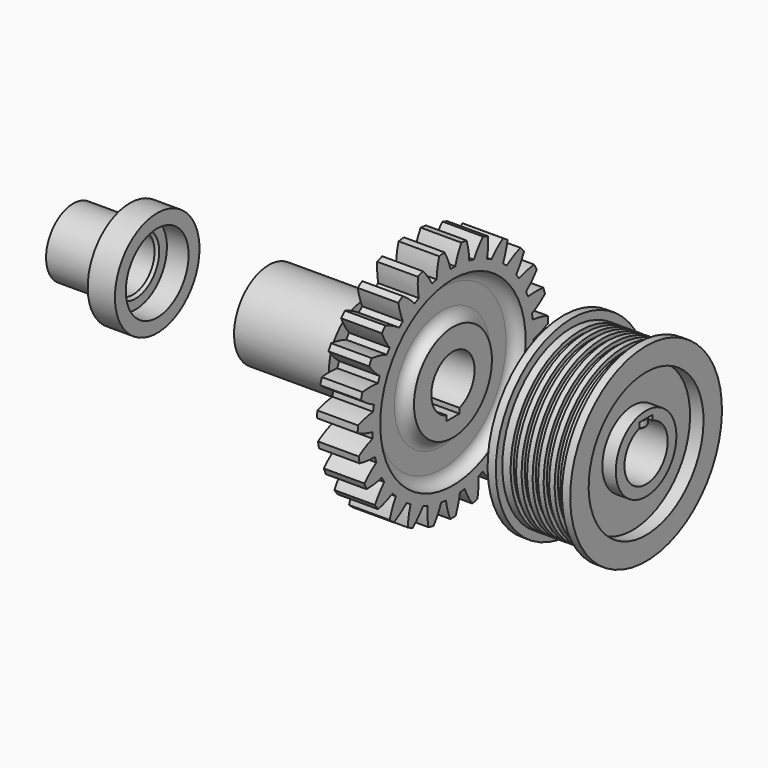
from build123d import *

# Parameters (mm, degrees)
F3_DEPTH  = 127
F7_DEPTH  = 45.212
F10_DEPTH = 39.878
F11_SIZE  = 2.032
F12_R     = 5.96899
F16_DEPTH = 33.02
F17_COUNT = 27
F17_ANGLE = 346.6666666667
F20_DEPTH = 33.02
F22_W     = 70.104
F22_H     = 12.065
F26_SIZE  = 1.905
F29_DEPTH = 6.096
F30_SIZE  = 0.762


# Not quite as in the source:
# - a fillet or chamfer that OpenCascade refuses, or shapes differently, is made with other operations: its cross-section is extruded or revolved along the edge and cut away or added
# - a fillet or chamfer is up to 0.001 mm smaller than in the source, because OpenCascade refuses the exact size


with BuildPart() as f1:
    # F0 (on Front) → F1 (revolve)
    with BuildSketch(Plane.XZ):
        Polygon((-30.48, 69.977), (-30.48, 52.959), (-20.574, 52.959), (-20.574, 27.94), (-30.48, 27.94), (-30.48, 19.939), (30.48, 19.939), (30.48, 27.94), (20.574, 27.94), (20.574, 52.959), (30.48, 52.959), (30.48, 69.977), (24.384, 69.977), (24.384, 64.008), (18.288, 64.008), (18.288, 60.96), (14.224, 60.96), (14.224, 64.008), (10.16, 64.008), (10.16, 60.96), (6.096, 60.96), (6.096, 64.008), (2.032, 64.008), (2.032, 60.96), (-2.032, 60.96), (-2.032, 64.008), (-6.096, 64.008), (-6.096, 60.96), (-10.16, 60.96), (-10.16, 64.008), (-14.224, 64.008), (-14.224, 60.96), (-18.288, 60.96), (-18.288, 64.008), (-24.384, 64.008), (-24.384, 69.977), align=None)
    revolve(axis=Axis((0, 0, 0), (1, 0, 0)))

    # F2 (on face) → F3 (cut)
    with BuildSketch(Plane(origin=(-30.48, 0, 0), x_dir=(0, -1, 0), z_dir=(-1, 0, 0))):
        with BuildLine():
            Line((5.969, 22.8345830441), (-5.969, 22.8345830441))
            Line((-5.969, 22.8345830441), (-5.969, 19.0245830441))
            ThreePointArc((-5.969, 19.0245830441), (0, 19.939), (5.969, 19.0245830441))
            Line((5.969, 19.0245830441), (5.969, 22.8345830441))
        make_face()
    extrude(amount=-F3_DEPTH, mode=Mode.SUBTRACT)


with BuildPart() as f5:
    # F4 (on Front) → F5 (revolve)
    with BuildSketch(Plane.XZ):
        Polygon((623.316, 19.939), (43.18, 19.939), (43.18, 0), (1083.056, 0), (1083.056, 19.939), (1003.3, 19.939), (1003.3, 28.956), (988.314, 28.956), (988.314, 19.939), (638.302, 19.939), (638.302, 28.956), (623.316, 28.956), align=None)
    revolve(axis=Axis((563.118, 0, 0), (1, 0, 0)))

    # F6 (on face) → F7 (cut)
    with BuildSketch(Plane(origin=(43.18, 0, 0), x_dir=(0, -1, 0), z_dir=(-1, 0, 0))):
        with BuildLine():
            ThreePointArc((5.969, 19.0245830441), (0, 19.939), (-5.969, 19.0245830441))
            Line((-5.969, 19.0245830441), (-5.969, 16.4845830441))
            Line((-5.969, 16.4845830441), (5.969, 16.4845830441))
            Line((5.969, 16.4845830441), (5.969, 19.0245830441))
        make_face()
    extrude(amount=-F7_DEPTH, mode=Mode.SUBTRACT)

    # F9 (on offset) → F10 (cut)
    with BuildSketch(Plane(origin=(585.216, 0, 0), x_dir=(0, -1, 0), z_dir=(-1, 0, 0))):
        with BuildLine():
            ThreePointArc((5.969, 19.0245830441), (0, 19.939), (-5.969, 19.0245830441))
            Line((-5.969, 19.0245830441), (-5.969, 16.4845830441))
            Line((-5.969, 16.4845830441), (5.969, 16.4845830441))
            Line((5.969, 16.4845830441), (5.969, 19.0245830441))
        make_face()
    extrude(amount=F10_DEPTH, mode=Mode.SUBTRACT)

    # F11
    f11_edges = [f5.edges().sort_by_distance(p)[0] for p in [
        (43.18, 0, -19.939),
        (1083.056, 0, -19.939),
    ]]
    chamfer(f11_edges, length=F11_SIZE)

    # F12 (radius 5.969 in the source; OpenCascade refuses exactly that, so slightly less here)
    f12_edges = [f5.edges().sort_by_distance(p)[0] for p in [
        (585.216, 5.969, 17.754583),
        (585.216, -5.969, 17.754583),
        (545.338, 5.969, 17.754583),
        (545.338, -5.969, 17.754583),
        (88.392, 5.969, 17.754583),
        (88.392, -5.969, 17.754583),
    ]]
    fillet(f12_edges, radius=F12_R)


with BuildPart() as f14:
    # F13 (on Front) → F14 (revolve)
    with BuildSketch(Plane.XZ):
        Polygon((-141.986, 35.941), (-141.986, 19.939), (-112.014, 19.939), (-112.014, 35.941), (-120.015, 35.941), (-120.015, 67.056), (-112.014, 67.056), (-112.014, 87.884), (-141.986, 87.884), (-141.986, 67.056), (-133.985, 67.056), (-133.985, 35.941), align=None)
    revolve(axis=Axis((-127, 0, 0), (1, 0, 0)))


with BuildPart() as f16:
    # F15 (on face) → F16 (new body)
    with BuildSketch(Plane(origin=(-141.986, 0, 0), x_dir=(0, -1, 0), z_dir=(-1, 0, 0))):
        with BuildLine():
            ThreePointArc((-7.747, 87.5418839585), (-4.5366280447, 81.1431985003), (-2.159, 74.3906768554))
            ThreePointArc((-2.159, 74.3906768554), (0, 74.422), (2.159, 74.3906768554))
            ThreePointArc((2.159, 74.3906768554), (4.5366280447, 81.1431985003), (7.747, 87.5418839585))
            ThreePointArc((7.747, 87.5418839585), (0, 87.884), (-7.747, 87.5418839585))
        make_face()
    extrude(amount=-F16_DEPTH)


with BuildPart() as f17_1:
    # F17: instance of F16
    add(f16.part.rotate(Axis((-141.986, 0, 0), (1, 0, 0)), 1 * F17_ANGLE / (F17_COUNT - 1)))


with BuildPart() as f17_2:
    # F17: instance of F16
    add(f16.part.rotate(Axis((-141.986, 0, 0), (1, 0, 0)), 2 * F17_ANGLE / (F17_COUNT - 1)))


with BuildPart() as f17_3:
    # F17: instance of F16
    add(f16.part.rotate(Axis((-141.986, 0, 0), (1, 0, 0)), 3 * F17_ANGLE / (F17_COUNT - 1)))


with BuildPart() as f17_4:
    # F17: instance of F16
    add(f16.part.rotate(Axis((-141.986, 0, 0), (1, 0, 0)), 4 * F17_ANGLE / (F17_COUNT - 1)))


with BuildPart() as f17_5:
    # F17: instance of F16
    add(f16.part.rotate(Axis((-141.986, 0, 0), (1, 0, 0)), 5 * F17_ANGLE / (F17_COUNT - 1)))


with BuildPart() as f17_6:
    # F17: instance of F16
    add(f16.part.rotate(Axis((-141.986, 0, 0), (1, 0, 0)), 6 * F17_ANGLE / (F17_COUNT - 1)))


with BuildPart() as f17_7:
    # F17: instance of F16
    add(f16.part.rotate(Axis((-141.986, 0, 0), (1, 0, 0)), 7 * F17_ANGLE / (F17_COUNT - 1)))


with BuildPart() as f17_8:
    # F17: instance of F16
    add(f16.part.rotate(Axis((-141.986, 0, 0), (1, 0, 0)), 8 * F17_ANGLE / (F17_COUNT - 1)))


with BuildPart() as f17_9:
    # F17: instance of F16
    add(f16.part.rotate(Axis((-141.986, 0, 0), (1, 0, 0)), 9 * F17_ANGLE / (F17_COUNT - 1)))


with BuildPart() as f17_10:
    # F17: instance of F16
    add(f16.part.rotate(Axis((-141.986, 0, 0), (1, 0, 0)), 10 * F17_ANGLE / (F17_COUNT - 1)))


with BuildPart() as f17_11:
    # F17: instance of F16
    add(f16.part.rotate(Axis((-141.986, 0, 0), (1, 0, 0)), 11 * F17_ANGLE / (F17_COUNT - 1)))


with BuildPart() as f17_12:
    # F17: instance of F16
    add(f16.part.rotate(Axis((-141.986, 0, 0), (1, 0, 0)), 12 * F17_ANGLE / (F17_COUNT - 1)))


with BuildPart() as f17_13:
    # F17: instance of F16
    add(f16.part.rotate(Axis((-141.986, 0, 0), (1, 0, 0)), 13 * F17_ANGLE / (F17_COUNT - 1)))


with BuildPart() as f17_14:
    # F17: instance of F16
    add(f16.part.rotate(Axis((-141.986, 0, 0), (1, 0, 0)), 14 * F17_ANGLE / (F17_COUNT - 1)))


with BuildPart() as f17_15:
    # F17: instance of F16
    add(f16.part.rotate(Axis((-141.986, 0, 0), (1, 0, 0)), 15 * F17_ANGLE / (F17_COUNT - 1)))


with BuildPart() as f17_16:
    # F17: instance of F16
    add(f16.part.rotate(Axis((-141.986, 0, 0), (1, 0, 0)), 16 * F17_ANGLE / (F17_COUNT - 1)))


with BuildPart() as f17_17:
    # F17: instance of F16
    add(f16.part.rotate(Axis((-141.986, 0, 0), (1, 0, 0)), 17 * F17_ANGLE / (F17_COUNT - 1)))


with BuildPart() as f17_18:
    # F17: instance of F16
    add(f16.part.rotate(Axis((-141.986, 0, 0), (1, 0, 0)), 18 * F17_ANGLE / (F17_COUNT - 1)))


with BuildPart() as f17_19:
    # F17: instance of F16
    add(f16.part.rotate(Axis((-141.986, 0, 0), (1, 0, 0)), 19 * F17_ANGLE / (F17_COUNT - 1)))


with BuildPart() as f17_20:
    # F17: instance of F16
    add(f16.part.rotate(Axis((-141.986, 0, 0), (1, 0, 0)), 20 * F17_ANGLE / (F17_COUNT - 1)))


with BuildPart() as f17_21:
    # F17: instance of F16
    add(f16.part.rotate(Axis((-141.986, 0, 0), (1, 0, 0)), 21 * F17_ANGLE / (F17_COUNT - 1)))


with BuildPart() as f17_22:
    # F17: instance of F16
    add(f16.part.rotate(Axis((-141.986, 0, 0), (1, 0, 0)), 22 * F17_ANGLE / (F17_COUNT - 1)))


with BuildPart() as f17_23:
    # F17: instance of F16
    add(f16.part.rotate(Axis((-141.986, 0, 0), (1, 0, 0)), 23 * F17_ANGLE / (F17_COUNT - 1)))


with BuildPart() as f17_24:
    # F17: instance of F16
    add(f16.part.rotate(Axis((-141.986, 0, 0), (1, 0, 0)), 24 * F17_ANGLE / (F17_COUNT - 1)))


with BuildPart() as f17_25:
    # F17: instance of F16
    add(f16.part.rotate(Axis((-141.986, 0, 0), (1, 0, 0)), 25 * F17_ANGLE / (F17_COUNT - 1)))


with BuildPart() as f17_26:
    # F17: instance of F16
    add(f16.part.rotate(Axis((-141.986, 0, 0), (1, 0, 0)), 26 * F17_ANGLE / (F17_COUNT - 1)))


with BuildPart() as f14_1:
    add(f14.part)

    # F18: cut F17_26, F16, F17_1, F17_2, F17_3, F17_4, F17_5, F17_6, F17_7, F17_8, F17_25, F17_9, F17_10, F17_11, F17_12, F17_13, F17_14, F17_15, F17_16, F17_17, F17_18, F17_19, F17_20, F17_21, F17_22, F17_23, F17_24
    add(f17_26.part, mode=Mode.SUBTRACT)
    add(f16.part, mode=Mode.SUBTRACT)
    add(f17_1.part, mode=Mode.SUBTRACT)
    add(f17_2.part, mode=Mode.SUBTRACT)
    add(f17_3.part, mode=Mode.SUBTRACT)
    add(f17_4.part, mode=Mode.SUBTRACT)
    add(f17_5.part, mode=Mode.SUBTRACT)
    add(f17_6.part, mode=Mode.SUBTRACT)
    add(f17_7.part, mode=Mode.SUBTRACT)
    add(f17_8.part, mode=Mode.SUBTRACT)
    add(f17_25.part, mode=Mode.SUBTRACT)
    add(f17_9.part, mode=Mode.SUBTRACT)
    add(f17_10.part, mode=Mode.SUBTRACT)
    add(f17_11.part, mode=Mode.SUBTRACT)
    add(f17_12.part, mode=Mode.SUBTRACT)
    add(f17_13.part, mode=Mode.SUBTRACT)
    add(f17_14.part, mode=Mode.SUBTRACT)
    add(f17_15.part, mode=Mode.SUBTRACT)
    add(f17_16.part, mode=Mode.SUBTRACT)
    add(f17_17.part, mode=Mode.SUBTRACT)
    add(f17_18.part, mode=Mode.SUBTRACT)
    add(f17_19.part, mode=Mode.SUBTRACT)
    add(f17_20.part, mode=Mode.SUBTRACT)
    add(f17_21.part, mode=Mode.SUBTRACT)
    add(f17_22.part, mode=Mode.SUBTRACT)
    add(f17_23.part, mode=Mode.SUBTRACT)
    add(f17_24.part, mode=Mode.SUBTRACT)

    # F19 (on face) → F20 (cut)
    with BuildSketch(Plane(origin=(-141.986, 0, 0), x_dir=(0, -1, 0), z_dir=(-1, 0, 0))):
        with BuildLine():
            ThreePointArc((5.969, -19.0245830441), (0, -19.939), (-5.969, -19.0245830441))
            Line((-5.969, -19.0245830441), (-5.969, -22.8345830441))
            Line((-5.969, -22.8345830441), (5.969, -22.8345830441))
            Line((5.969, -22.8345830441), (5.969, -19.0245830441))
        make_face()
    extrude(amount=-F20_DEPTH, mode=Mode.SUBTRACT)

    # F21: fillet of radius 8.128 on 4 edges, made by hand


with BuildPart() as f21_tool2:
    # F21_s3 → F21_t4 (revolve)
    with BuildSketch(Plane.XZ):
        with BuildLine():
            ThreePointArc((-133.985, 44.069), (-136.3656360825, 38.3216360825), (-142.113, 35.941))
            Line((-142.113, 35.941), (-133.985, 35.941))
            Line((-133.985, 35.941), (-133.985, 44.069))
        make_face()
    revolve(axis=Axis((-133.985, 0, 0), (1, 0, 0)))

    split(bisect_by=Plane.YZ.offset(-141.986), keep=Keep.TOP)


with BuildPart() as f14_2:
    add(f14_1.part)

    # F21_t1: union F21_tool2
    add(f21_tool2.part)


with BuildPart() as f21_tool7:
    # F21_s8 → F21_t9 (revolve)
    with BuildSketch(Plane.XZ):
        with BuildLine():
            ThreePointArc((-142.113, 67.056), (-136.3656360825, 64.6753639175), (-133.985, 58.928))
            Line((-133.985, 58.928), (-133.985, 67.056))
            Line((-133.985, 67.056), (-142.113, 67.056))
        make_face()
    revolve(axis=Axis((-133.985, 0, 0), (1, 0, 0)))

    split(bisect_by=Plane.YZ.offset(-141.986), keep=Keep.TOP)


with BuildPart() as f14_3:
    add(f14_2.part)

    # F21_t6: union F21_tool7
    add(f21_tool7.part)


with BuildPart() as f21_tool12:
    # F21_s13 → F21_t14 (revolve)
    with BuildSketch(Plane.XZ):
        with BuildLine():
            ThreePointArc((-111.887, 35.941), (-117.6343639175, 38.3216360825), (-120.015, 44.069))
            Line((-120.015, 44.069), (-120.015, 35.941))
            Line((-120.015, 35.941), (-111.887, 35.941))
        make_face()
    revolve(axis=Axis((-120.015, 0, 0), (1, 0, 0)))

    split(bisect_by=Plane.YZ.offset(-112.014), keep=Keep.BOTTOM)


with BuildPart() as f14_4:
    add(f14_3.part)

    # F21_t11: union F21_tool12
    add(f21_tool12.part)


with BuildPart() as f21_tool17:
    # F21_s18 → F21_t19 (revolve)
    with BuildSketch(Plane.XZ):
        with BuildLine():
            ThreePointArc((-120.015, 58.928), (-117.6343639175, 64.6753639175), (-111.887, 67.056))
            Line((-111.887, 67.056), (-120.015, 67.056))
            Line((-120.015, 67.056), (-120.015, 58.928))
        make_face()
    revolve(axis=Axis((-120.015, 0, 0), (1, 0, 0)))

    split(bisect_by=Plane.YZ.offset(-112.014), keep=Keep.BOTTOM)


with BuildPart() as f14_5:
    add(f14_4.part)

    # F21_t16: union F21_tool17
    add(f21_tool17.part)


with BuildPart() as f23:
    # F22 (on Front) → F23 (revolve)
    with BuildSketch(Plane.XZ):
        with Locations((-212.852, 25.9715)):
            Rectangle(F22_W, F22_H)
    revolve(axis=Axis((-212.852, 0, 0), (-1, 0, 0)))


with BuildPart() as f25:
    # F24 (on Front) → F25 (revolve)
    with BuildSketch(Plane.XZ):
        Polygon((-392.176, 25.019), (-392.176, 19.939), (-346.202, 19.939), (-346.202, 28.956), (-330.2, 28.956), (-330.2, 38.989), (-350.266, 38.989), (-350.266, 25.019), align=None)
    revolve(axis=Axis((-361.188, 0, 0), (1, 0, 0)))

    # F26
    f26_edges = [f25.edges().sort_by_distance(p)[0] for p in [
        (-392.176, 0, -19.939),
        (-346.202, 0, -19.939),
    ]]
    chamfer(f26_edges, length=F26_SIZE)


with BuildPart() as f29:
    # F28 (on face) → F29 (new body)
    with BuildSketch(Plane(origin=(0, 0, 22.8345830441), x_dir=(1, 0, 0), z_dir=(0, 0, -1))):
        with BuildLine():
            ThreePointArc((24.13, -5.969), (30.099, 0), (24.13, 5.969))
            Line((24.13, 5.969), (8.128, 5.969))
            ThreePointArc((8.128, 5.969), (2.159, 0), (8.128, -5.969))
            Line((8.128, -5.969), (24.13, -5.969))
        make_face()
    extrude(amount=F29_DEPTH)

    # F30
    f30_edges = [f29.edges().sort_by_distance(p)[0] for p in [
        (16.129, -5.969, 16.738583),
        (16.129, -5.969, 22.834583),
    ]]
    chamfer(f30_edges, length=F30_SIZE)


solid = Compound([f1.part, f14_5.part, f23.part, f25.part, f29.part])
